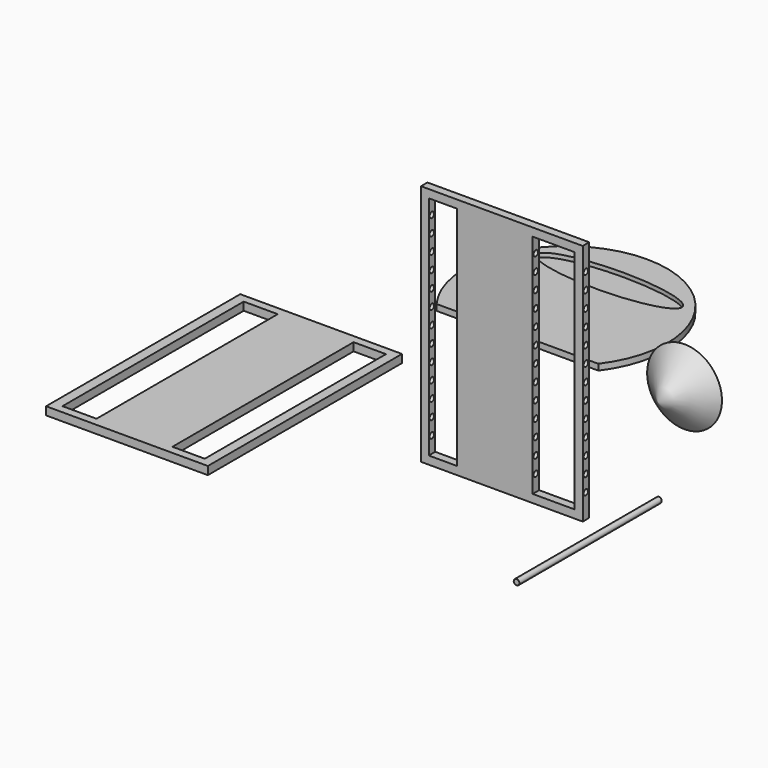
from build123d import *

# Parameters (mm, degrees)
F0_W      = 88.1795883179
F0_H      = 711.2
F1_DEPTH  = 25.4
F3_DEPTH  = 19.05
F4_R      = 8.89
F5_DEPTH  = 564.8227298821
F8_R      = 8.89
F9_DEPTH  = 558.8
F11_DEPTH = 25.4
F12_DEPTH = 6.35


# Not quite as in the source:
# - a feature names something its author has since deleted; it is built from what else it names


with BuildPart() as f1:
    # F0 (on Front) → F1 (new body)
    with BuildSketch(Plane.XZ):
        Polygon((-402.5202535568, 375.1774401814), (-402.5202535568, -386.8225598186), (80.0489783287, -386.8225598186), (80.0489783287, -361.4225598186), (-51.7384251099, -361.4225598186), (-51.7384251099, 349.7774401814), (-51.7384251099, 375.1774401814), align=None)
        with Locations((-334.0802192688, -5.8225598186)):
            Rectangle(F0_W, F0_H, mode=Mode.SUBTRACT)
        Polygon((80.0489783287, -361.4225598186), (80.0489783287, -386.8225598186), (105.4797464432, -386.8225598186), (105.4797464432, 375.1774401814), (-51.7384251099, 375.1774401814), (-51.7384251099, 349.7774401814), (80.0489783287, 349.7774401814), align=None)
    extrude(amount=F1_DEPTH)

    # F4 (on face) → F5 (cut, through all)
    with BuildSketch(Plane(origin=(-402.5202535568, 0, 0), x_dir=(0, -1, 0), z_dir=(-1, 0, 0))):
        with Locations((13.0486593567, -310.6189571056)):
            Circle(F4_R)
        with Locations((13.0486593567, -259.8189571056)):
            Circle(F4_R)
        with Locations((13.0486593567, -209.0189571056)):
            Circle(F4_R)
        with Locations((13.0486593567, 146.5810428944)):
            Circle(F4_R)
        with Locations((13.0486593567, 95.7810428944)):
            Circle(F4_R)
        with Locations((13.0486593567, 44.9810428944)):
            Circle(F4_R)
        with Locations((13.0486593567, -5.8189571056)):
            Circle(F4_R)
        with Locations((13.0486593567, -56.6189571056)):
            Circle(F4_R)
        with Locations((13.0486593567, -107.4189571056)):
            Circle(F4_R)
        with Locations((13.0486593567, -158.2189571056)):
            Circle(F4_R)
        with Locations((13.0491397289, 298.9786399844)):
            Circle(F4_R)
        with Locations((13.3982794578, 248.1798397875)):
            Circle(F4_R)
        with Locations((13.0486593567, 197.3810428944)):
            Circle(F4_R)
    extrude(amount=-F5_DEPTH, mode=Mode.SUBTRACT)


with BuildPart() as f3:
    # F2 (on Top) → F3 (new body)
    with BuildSketch(Plane.XY):
        with BuildLine():
            ThreePointArc((-155.1985237747, 552.16276142), (-439.1791569172, 376.6530779912), (-409.1985237747, 44.16276142))
            Line((-409.1985237747, 44.16276142), (-155.1985237747, 44.16276142))
            Line((-155.1985237747, 44.16276142), (-155.1985237747, 351.4989493568))
            add(Edge.make_bspline(
                [(-155.1985237747, 460.6216074745), (-381.9626234472, 460.6216074745), (-381.9626234472, 406.0602784157), (-381.9626234472, 351.4989493568), (-155.1985237747, 351.4989493568)],
                knots=[1.5707963268, 1.5707963268, 1.5707963268, 3.1415926536, 3.1415926536, 4.7123889804, 4.7123889804, 4.7123889804], degree=2, weights=[1, 0.7071067812, 1, 0.7071067812, 1]))
            Line((-155.1985237747, 460.6216074745), (-155.1985237747, 552.16276142))
        make_face()
        with BuildLine():
            Line((-155.1985237747, 351.4989493568), (-155.1985237747, 44.16276142))
            Line((-155.1985237747, 44.16276142), (98.8014762253, 44.16276142))
            ThreePointArc((98.8014762253, 44.16276142), (128.7821093677, 376.6530779912), (-155.1985237747, 552.16276142))
            Line((-155.1985237747, 552.16276142), (-155.1985237747, 460.6216074745))
            add(Edge.make_bspline(
                [(71.5655758977, 406.0602784157), (71.5655758977, 460.6216074745), (-155.1985237747, 460.6216074745)],
                knots=[0, 0, 0, 1.5707963268, 1.5707963268, 1.5707963268], degree=2, weights=[1, 0.7071067812, 1]))
            add(Edge.make_bspline(
                [(-155.1985237747, 351.4989493568), (71.5655758977, 351.4989493568), (71.5655758977, 406.0602784157)],
                knots=[4.7123889804, 4.7123889804, 4.7123889804, 6.2831853072, 6.2831853072, 6.2831853072], degree=2, weights=[1, 0.7071067812, 1]))
        make_face()
    extrude(amount=F3_DEPTH)

    # F2 (on Top) → F12 (join)
    with BuildSketch(Plane.XY):
        with BuildLine():
            add(Edge.make_bspline(
                [(-155.1985237747, 460.6216074745), (-381.9626234472, 460.6216074745), (-381.9626234472, 406.0602784157), (-381.9626234472, 351.4989493568), (-155.1985237747, 351.4989493568)],
                knots=[1.5707963268, 1.5707963268, 1.5707963268, 3.1415926536, 3.1415926536, 4.7123889804, 4.7123889804, 4.7123889804], degree=2, weights=[1, 0.7071067812, 1, 0.7071067812, 1]))
            Line((-155.1985237747, 351.4989493568), (-155.1985237747, 460.6216074745))
        make_face()
        with BuildLine():
            Line((-155.1985237747, 460.6216074745), (-155.1985237747, 351.4989493568))
            add(Edge.make_bspline(
                [(-155.1985237747, 351.4989493568), (71.5655758977, 351.4989493568), (71.5655758977, 406.0602784157)],
                knots=[4.7123889804, 4.7123889804, 4.7123889804, 6.2831853072, 6.2831853072, 6.2831853072], degree=2, weights=[1, 0.7071067812, 1]))
            add(Edge.make_bspline(
                [(71.5655758977, 406.0602784157), (71.5655758977, 460.6216074745), (-155.1985237747, 460.6216074745)],
                knots=[0, 0, 0, 1.5707963268, 1.5707963268, 1.5707963268], degree=2, weights=[1, 0.7071067812, 1]))
        make_face()
    extrude(amount=F12_DEPTH)


with BuildPart() as f7:
    # F6 (on Top) → F7 (revolve)
    with BuildSketch(Plane.XY):
        Polygon((317.2058165073, 109.4450652599), (199.6315717697, 109.4450652599), (317.2058165073, 5.5246124975), align=None)
    revolve(axis=Axis((317.2058165073, 57.4848388787, 0), (0, -1, 0)))


with BuildPart() as f9:
    # F8 (on Front) → F9 (new body)
    with BuildSketch(Plane.XZ):
        with Locations((324.3089020252, -266.2139832973)):
            Circle(F8_R)
    extrude(amount=F9_DEPTH)


with BuildPart() as f11:
    # F10 (on Top) → F11 (new body)
    with BuildSketch(Plane.XY):
        Polygon((-754.7940611839, -187.2776719332), (-840.7245906978, -187.2776719332), (-840.7245906978, -949.2776719332), (-332.7245906978, -949.2776719332), (-332.7245906978, -187.2776719332), (-426.6838133335, -187.2776719332), (-426.6838133335, -212.6776719332), (-362.7426974754, -212.6776719332), (-362.7426974754, -923.8776719332), (-464.3426974754, -923.8776719332), (-464.3426974754, -212.6776719332), (-702.5946974754, -212.6776719332), (-702.5946974754, -923.8776719332), (-809.4791173935, -923.8776719332), (-809.4791173935, -212.6776719332), (-754.7940611839, -212.6776719332), align=None)
        Polygon((-426.6838133335, -187.2776719332), (-754.7940611839, -187.2776719332), (-754.7940611839, -212.6776719332), (-702.5946974754, -212.6776719332), (-464.3426974754, -212.6776719332), (-426.6838133335, -212.6776719332), align=None)
    extrude(amount=-F11_DEPTH)


solid = Compound([f1.part, f3.part, f7.part, f9.part, f11.part])
